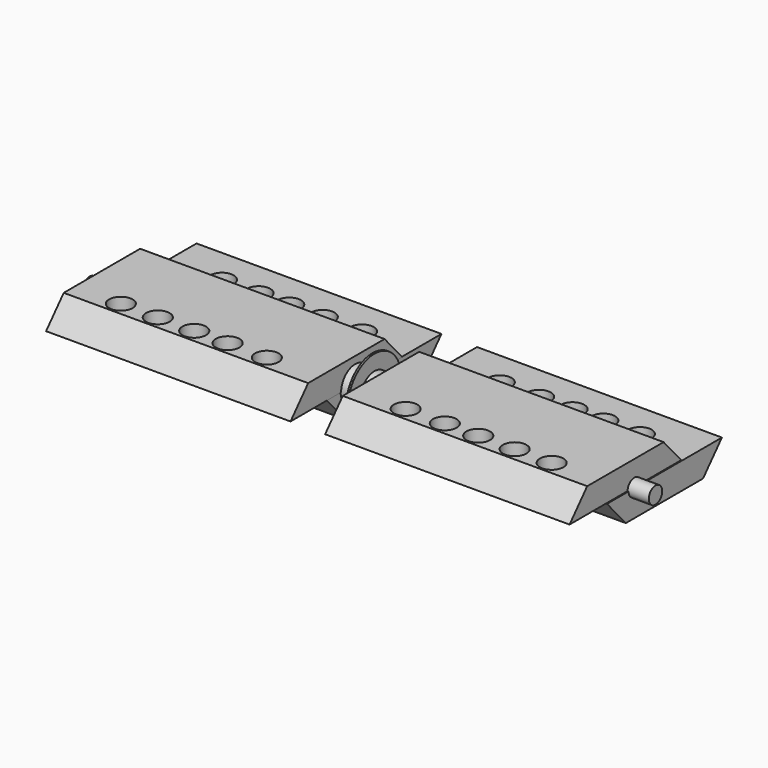
from build123d import *

# Parameters (mm, degrees)
F1_DEPTH     = 152.4
F4_W         = 131.646358408
F4_H         = 76.841160655
F5_DEPTH     = 13.3604
F6_T1_DEPTH  = 205.2440690488
F7_T1_DEPTH  = 205.2440690488
F9_DEPTH     = 14.2875
F10_T1_DEPTH = 205.504029119
F10_T6_DEPTH = 205.504029119
F13_D        = 12.7
F15_D        = 12.7
F15_DEPTH    = 13.3614
F17_R        = 9.525
F18_DEPTH    = 25.4
F20_R        = 17.78
F21_DEPTH    = 1.016


# Not quite as in the source:
# - a fillet or chamfer that OpenCascade refuses, or shapes differently, is made with other operations: its cross-section is extruded or revolved along the edge and cut away or added
# - two fillets or chamfers of one size are made in one step
# - a feature names something its author has since deleted; it is built from what else it names


with BuildPart() as f1:
    # F0 (on Right) → F1 (new body)
    with BuildSketch(Plane.YZ):
        with BuildLine():
            ThreePointArc((1.0781578021, -4.3934942223), (3.559679728, -2.7917549967), (4.523849658, 0))
            ThreePointArc((4.523849658, 0), (-3.559679728, 2.7917549967), (1.0781578021, -4.3934942223))
        make_face()
    extrude(amount=F1_DEPTH)

    # F4 (on Top) → F5 (join)
    with BuildSketch(Plane.XY):
        with Locations((75.142014306, -5.9899426997)):
            Rectangle(F4_W, F4_H)
    extrude(amount=F5_DEPTH)

    # F6: chamfer of 12.7 x 14.2875 on 1 edges, made by hand

    # F6_s2 → F6_t1 (cut)
    with BuildSketch(Plane.YZ.offset(-27.4800202183)):
        Polygon((-44.4105230272, -0.9271), (-31.7105230272, 13.3604), (-44.4105230272, 13.3604), align=None)
    extrude(amount=F6_T1_DEPTH, mode=Mode.SUBTRACT)

    # F7: chamfer of 14.2875 x 12.7 on 1 edges, made by hand

    # F7_s2 → F7_t1 (cut)
    with BuildSketch(Plane.YZ.offset(-27.4800202183)):
        Polygon((19.7306376278, 13.3604), (32.4306376278, -0.9271), (32.4306376278, 13.3604), align=None)
    extrude(amount=F7_T1_DEPTH, mode=Mode.SUBTRACT)

    # F8 (on Top) → F9 (join)
    with BuildSketch(Plane.XY):
        Polygon((9.5707597211, 58.3520196378), (9.5707597211, 0), (9.5707597211, -19.05), (141.4770781994, -19.05), (141.4770781994, 58.3520196378), align=None)
    extrude(amount=-F9_DEPTH)

    # F10: chamfer of 12.7 x 14.2875 on 2 edges, made by hand

    # F10_s2 → F10_t1 (cut)
    with BuildSketch(Plane.YZ.offset(-27.2280955993)):
        Polygon((45.6520196378, -14.2875), (58.3520196378, 0), (58.3520196378, -14.2875), align=None)
    extrude(amount=F10_T1_DEPTH, mode=Mode.SUBTRACT)


with BuildPart() as f10_tool4:
    # F10_s5 → F10_t6 (new body)
    with BuildSketch(Plane.YZ.offset(-27.2280955993)):
        Polygon((-19.05, 0), (-6.35, -14.2875), (-19.05, -14.2875), align=None)
    extrude(amount=F10_T6_DEPTH)

    split(bisect_by=Plane.XY, keep=Keep.BOTTOM)


with BuildPart() as f1_1:
    add(f1.part)

    # F10_t3: cut F10_tool4
    add(f10_tool4.part, mode=Mode.SUBTRACT)

    # F13 (through all)
    with Locations(Plane.XY):
        with Locations((76.2983709574, 39.286326617), (92.8492099047, 39.286326617), (112.5427857041, 39.286326617), (58.2417622209, 39.286326617), (37.0924063027, 39.286326617)):
            Hole(F13_D / 2)

    # F15 (through all, one way)
    with BuildSketch(Plane(origin=(0, 0, 0), x_dir=(1, 0, 0), z_dir=(0, 0, -1))):
        with Locations((116.0114407539, 24.4592092931), (96.1036607623, 24.4592092931), (76.4752775431, 24.4592092931), (37.3658165336, 24.4592092931), (58.4825836122, 24.4592092931)):
            Circle(F15_D / 2)
    extrude(amount=-F15_DEPTH, mode=Mode.SUBTRACT)

    # F16: F1 across plane


with BuildPart() as f1_2:
    add(f1_1.part)
    add(f1_1.part.mirror(Plane.YZ))

    # F17 (on Right) → F18 (join)
    with BuildSketch(Plane.YZ):
        Circle(F17_R)
    extrude(amount=F18_DEPTH)


with BuildPart() as f19_1:
    # F19: instance of F1
    add(f1_2.part.mirror(Plane.YZ))


with BuildPart() as f21:
    # F20 (on Right) → F21 (new body)
    with BuildSketch(Plane.YZ):
        Circle(F20_R)
    extrude(amount=F21_DEPTH)


solid = Compound([f1_2.part, f19_1.part, f21.part])
